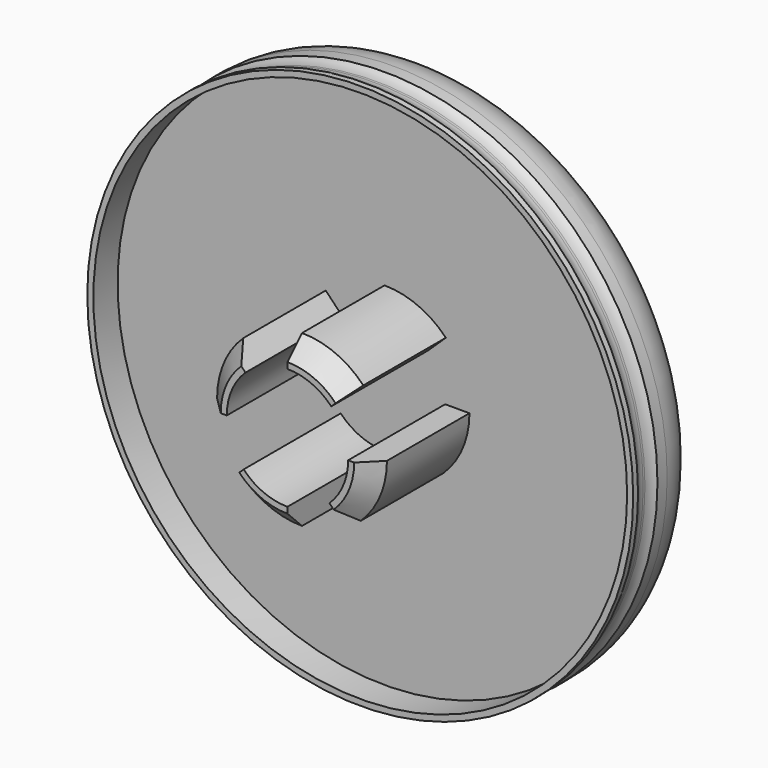
from build123d import *

# Parameters (mm, degrees)
F0_R      = 57.15
F0_R_2    = 54.61
F1_DEPTH  = 12.7
F2_R      = 57.15
F2_R_2    = 55.88
F3_DEPTH  = 6.35
F5_DEPTH  = 25.4
F6_R      = 10.16
F8_R      = 57.3643246116
F8_R_2    = 56.3769302999
F9_DEPTH  = 5.08
F11_SIZE  = 3.81
F12_R     = 30.0710840357
F13_DEPTH = 5.08


# Not quite as in the source:
# - a fillet or chamfer that OpenCascade refuses, or shapes differently, is made with other operations: its cross-section is extruded or revolved along the edge and cut away or added
# - a feature names something its author has since deleted; it is built from what else it names


with BuildPart() as f1:
    # F0 (on Front) → F1 (new body)
    with BuildSketch(Plane.XZ):
        Circle(F0_R)
        Circle(F0_R_2, mode=Mode.SUBTRACT)
        Circle(F0_R_2)
    extrude(amount=F1_DEPTH)

    # F2 (on face) → F3 (join)
    with BuildSketch(Plane.XZ.offset(12.7)):
        Circle(F2_R)
        Circle(F2_R_2, mode=Mode.SUBTRACT)
    extrude(amount=F3_DEPTH)

    # F4 (on face) → F5 (join)
    with BuildSketch(Plane.XZ.offset(12.7)):
        with BuildLine():
            Line((9.1685925479, 8.7878843126), (12.836029567, 12.3030380376))
            ThreePointArc((12.836029567, 12.3030380376), (6.9778357566, 16.3535380928), (0, 17.78))
            Line((0, 17.78), (0, 12.7))
            ThreePointArc((0, 12.7), (4.9841683976, 11.6810986377), (9.1685925479, 8.7878843126))
        make_face()
        with BuildLine():
            ThreePointArc((12.3030380376, -12.836029567), (16.3535380928, -6.9778357566), (17.78, 0))
            Line((17.78, 0), (12.7, 0))
            ThreePointArc((12.7, 0), (11.6810986377, -4.9841683976), (8.7878843126, -9.1685925479))
            Line((8.7878843126, -9.1685925479), (12.3030380376, -12.836029567))
        make_face()
        with BuildLine():
            ThreePointArc((-12.836029567, -12.3030380376), (-6.9778357566, -16.3535380928), (0, -17.78))
            Line((0, -17.78), (0, -12.7))
            ThreePointArc((0, -12.7), (-4.9841683976, -11.6810986377), (-9.1685925479, -8.7878843126))
            Line((-9.1685925479, -8.7878843126), (-12.836029567, -12.3030380376))
        make_face()
        with BuildLine():
            Line((-8.7878843126, 9.1685925479), (-12.3030380376, 12.836029567))
            ThreePointArc((-12.3030380376, 12.836029567), (-16.3535380928, 6.9778357566), (-17.78, 0))
            Line((-17.78, 0), (-12.7, 0))
            ThreePointArc((-12.7, 0), (-11.6810986377, 4.9841683976), (-8.7878843126, 9.1685925479))
        make_face()
    extrude(amount=F5_DEPTH)

    # F6
    f6_edges = [f1.edges().sort_by_distance(p)[0] for p in [
        (-57.15, 0, 0),
    ]]
    fillet(f6_edges, radius=F6_R)

    # F8 (on offset) → F9 (cut)
    with BuildSketch(Plane.XZ.offset(12.7)):
        Circle(F8_R)
        Circle(F8_R_2, mode=Mode.SUBTRACT)
    extrude(amount=F9_DEPTH, mode=Mode.SUBTRACT)

    # F10: fillet of radius 3.81 on 3 edges, made by hand

    # F10_s1 → F10_t2 (revolve)
    with BuildSketch(Plane.XY):
        with BuildLine():
            ThreePointArc((56.3769302999, -15.0006856268), (56.5753652345, -13.7871380263), (57.15, -12.7))
            Line((57.15, -12.7), (57.089261394, -12.6539862875))
            ThreePointArc((57.089261394, -12.6539862875), (56.7634651499, -12.6238), (56.3769302999, -12.6238))
            Line((56.3769302999, -12.6238), (56.3007302999, -12.7))
            Line((56.3007302999, -12.7), (56.3007302999, -15.0006856268))
            Line((56.3007302999, -15.0006856268), (56.3769302999, -15.0006856268))
        make_face()
    revolve(axis=Axis((0, -12.7, 0), (0, -1, 0)))

    # F10_s3 → F10_t4 (revolve)
    with BuildSketch(Plane.XY):
        with BuildLine():
            ThreePointArc((57.15, -17.78), (56.5753652345, -16.6928619737), (56.3769302999, -15.4793143732))
            Line((56.3769302999, -15.4793143732), (56.3007302999, -15.4793143732))
            Line((56.3007302999, -15.4793143732), (56.3007302999, -17.78))
            Line((56.3007302999, -17.78), (56.3769302999, -17.8562))
            ThreePointArc((56.3769302999, -17.8562), (56.7634651499, -17.8562), (57.089261394, -17.8260137125))
            Line((57.089261394, -17.8260137125), (57.15, -17.78))
        make_face()
    revolve(axis=Axis((0, -17.78, 0), (0, -1, 0)))

    # F11
    f11_edges = [f1.edges().sort_by_distance(p)[0] for p in [
        (-16.353538, -38.1, 6.977836),
        (-6.977836, -38.1, -16.353538),
        (16.353538, -38.1, -6.977836),
        (6.977836, -38.1, 16.353538),
    ]]
    chamfer(f11_edges, length=F11_SIZE)

    # F12 (on face) → F13 (cut)
    with BuildSketch(Plane(origin=(0, 0, 0), x_dir=(-1, 0, 0), z_dir=(0, 1, 0))):
        Circle(F12_R)
    extrude(amount=-F13_DEPTH, mode=Mode.SUBTRACT)

    # F14: fillet of radius 86.36 on 1 edges, made by hand

    # F14_s1 → F14_t2 (revolve)
    with BuildSketch(Plane.XY):
        with BuildLine():
            ThreePointArc((-30.0710840357, 0), (-15.6993236042, -3.8005218602), (-0.8887057913, -5.08))
            Line((-0.8887057913, -5.08), (-30.0710840357, -5.08))
            Line((-30.0710840357, -5.08), (-30.0710840357, 0))
        make_face()
    revolve(axis=Axis((0, -5.08, 0), (0, 1, 0)))


solid = f1.part
